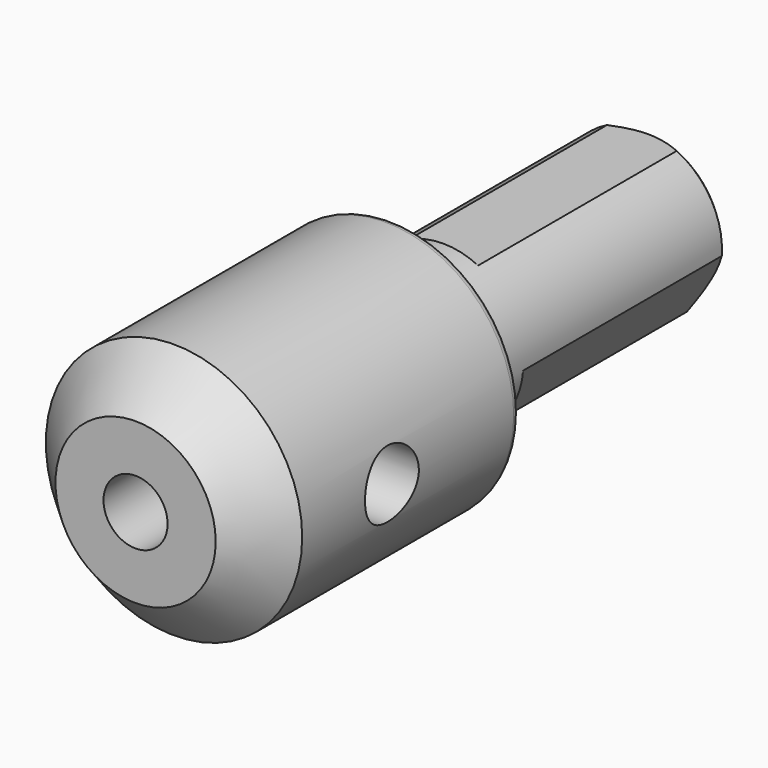
from build123d import *

# Parameters (mm, degrees)
F0_R            = 8
F1_DEPTH        = 20
F2_R            = 5
F3_DEPTH        = 20
F5_DEPTH        = 16
F5_COPIES_COUNT = 3
F6_SIZE         = 0.49999
F7_R            = 0.5
F9_D            = 4
F9_DEPTH        = 14
F9_TIP          = 1.2017212381
F10_R           = 2.1
F11_DEPTH       = 8.25
F12_SIZE        = 3


# Not quite as in the source:
# - a fillet or chamfer is up to 0.001 mm smaller than in the source, because OpenCascade refuses the exact size
# - a pattern or mirror of a feature is missing from the dataset's text; its kind, count and spacing are read off the source's solid


with BuildPart() as f1:
    # F0 (on Front) → F1 (new body)
    with BuildSketch(Plane.XZ):
        Circle(F0_R)
    extrude(amount=-F1_DEPTH)

    # F2 (on face) → F3 (join)
    with BuildSketch(Plane(origin=(0, 20, 0), x_dir=(-1, 0, 0), z_dir=(0, 1, 0))):
        Circle(F2_R)
    extrude(amount=F3_DEPTH)

    # F4 (on face) → F5 (cut)
    with BuildSketch(Plane(origin=(0, 40, 0), x_dir=(-1, 0, 0), z_dir=(0, 1, 0))):
        with BuildLine():
            ThreePointArc((2.1794494718, 4.5), (0, 5), (-2.1794494718, 4.5))
            Line((-2.1794494718, 4.5), (2.1794494718, 4.5))
        make_face()
    f5 = extrude(amount=-F5_DEPTH, mode=Mode.SUBTRACT)

    # F5_copies: F5 ×3 about axis
    f5_copies_axis = Axis((0, 0, 0), (0, 1, 0))
    for i in range(1, F5_COPIES_COUNT):
        add(f5.rotate(f5_copies_axis, i * 360 / F5_COPIES_COUNT), mode=Mode.SUBTRACT)

    # F6 (size 0.5 in the source; OpenCascade refuses exactly that, so slightly less here)
    f6_edges = [f1.edges().sort_by_distance(p)[0] for p in [
        (4.330127, 40, 2.5),
        (-4.996709, 40, -0.18139),
        (0, 40, -5),
        (-4.236582, 40, 2.655443),
    ]]
    chamfer(f6_edges, length=F6_SIZE)

    # F7
    f7_edges = [f1.edges().sort_by_distance(p)[0] for p in [
        (-8, 20, 0),
        (5, 20, 0),
    ]]
    fillet(f7_edges, radius=F7_R)

    # F9
    with Locations(Plane.XZ):
        with Locations((0, 0)):
            Hole(F9_D / 2, depth=F9_DEPTH)
            with Locations((0, 0, -(F9_DEPTH + F9_TIP / 2))):  # 118° drill point
                Cone(0, F9_D / 2, F9_TIP, mode=Mode.SUBTRACT)

    # F10 (on Right) → F11 (cut, symmetric)
    with BuildSketch(Plane.YZ):
        with Locations((10, 0)):
            Circle(F10_R)
    extrude(amount=F11_DEPTH, both=True, mode=Mode.SUBTRACT)

    # F12
    f12_edges = [f1.edges().sort_by_distance(p)[0] for p in [
        (-8, 0, 0),
    ]]
    chamfer(f12_edges, length=F12_SIZE)


solid = f1.part
